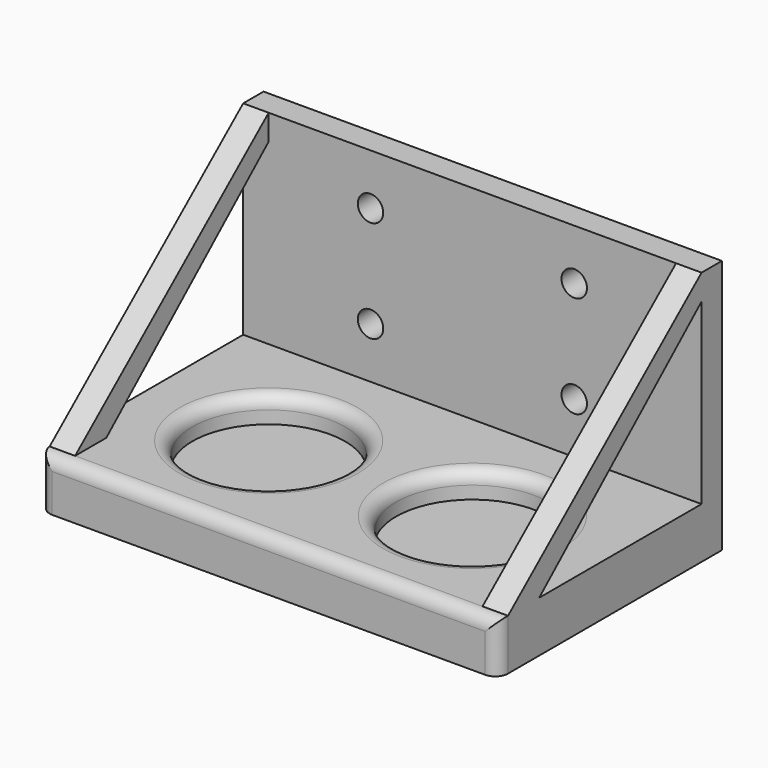
from build123d import *

# Parameters (mm, degrees)
F0_W      = 114.3
F0_H      = 63.5
F0_R      = 19.05
F1_DEPTH  = 12.7
F2_DEPTH  = 6.35
F3_W      = 6.35
F3_H      = 60.325
F4_DEPTH  = 50.8
F6_DEPTH  = 114.301
F7_W      = 101.6
F7_H      = 50.8
F7_R      = 3.175
F8_DEPTH  = 6.35
F9_R      = 3.17499
F11_DEPTH = 114.301


# Not quite as in the source:
# - a fillet or chamfer is up to 0.001 mm smaller than in the source, because OpenCascade refuses the exact size


with BuildPart() as f1:
    # F0 (on Top) → F1 (new body)
    with BuildSketch(Plane.XY):
        Rectangle(F0_W, F0_H)
        with Locations((-25.4, 0)):
            Circle(F0_R, mode=Mode.SUBTRACT)
        with Locations((25.4, 0)):
            Circle(F0_R, mode=Mode.SUBTRACT)
    extrude(amount=F1_DEPTH)

    # F0 (on Top) → F2 (join)
    with BuildSketch(Plane.XY):
        with Locations((-25.4, 0)):
            Circle(F0_R)
        with Locations((25.4, 0)):
            Circle(F0_R)
    extrude(amount=F2_DEPTH)

    # F3 (on face) → F4 (join)
    with BuildSketch(Plane.XY.offset(12.7)):
        with Locations((-53.975, 1.5875)):
            Rectangle(F3_W, F3_H)
        with Locations((53.975, 1.5875)):
            Rectangle(F3_W, F3_H)
    extrude(amount=F4_DEPTH)

    # F5 (on face) → F6 (cut, through all)
    with BuildSketch(Plane(origin=(-57.15, 0, 0), x_dir=(0, -1, 0), z_dir=(-1, 0, 0))):
        Polygon((28.575, 63.5), (-31.75, 63.5), (28.575, 12.7), align=None)
    extrude(amount=-F6_DEPTH, mode=Mode.SUBTRACT)

    # F7 (on face) → F8 (join)
    with BuildSketch(Plane(origin=(0, 31.75, 0), x_dir=(-1, 0, 0), z_dir=(0, 1, 0))):
        Polygon((-50.8, 12.7), (-50.8, 63.5), (-57.15, 63.5), (-57.15, 0), (57.15, 0), (57.15, 63.5), (50.8, 63.5), (50.8, 12.7), align=None)
        with Locations((0, 38.1)):
            Rectangle(F7_W, F7_H)
        with Locations((-25.4, 25.4)):
            Circle(F7_R, mode=Mode.SUBTRACT)
        with Locations((25.4, 25.4)):
            Circle(F7_R, mode=Mode.SUBTRACT)
        with Locations((-25.4, 50.8)):
            Circle(F7_R, mode=Mode.SUBTRACT)
        with Locations((25.4, 50.8)):
            Circle(F7_R, mode=Mode.SUBTRACT)
    extrude(amount=F8_DEPTH)

    # F9 (radius 3.175 in the source; OpenCascade refuses exactly that, so slightly less here)
    f9_edges = [f1.edges().sort_by_distance(p)[0] for p in [
        (-44.45, 0, 12.7),
        (6.35, 0, 12.7),
        (0, -31.75, 12.7),
        (57.15, -31.75, 6.35),
        (-57.15, -31.75, 6.35),
    ]]
    fillet(f9_edges, radius=F9_R)

    # F10 (on face) → F11 (cut, through all)
    with BuildSketch(Plane.YZ.offset(57.15)):
        Polygon((31.75, 12.7), (31.75, 57.15), (-18.8612597303, 12.7), align=None)
    extrude(amount=-F11_DEPTH, mode=Mode.SUBTRACT)


solid = f1.part
